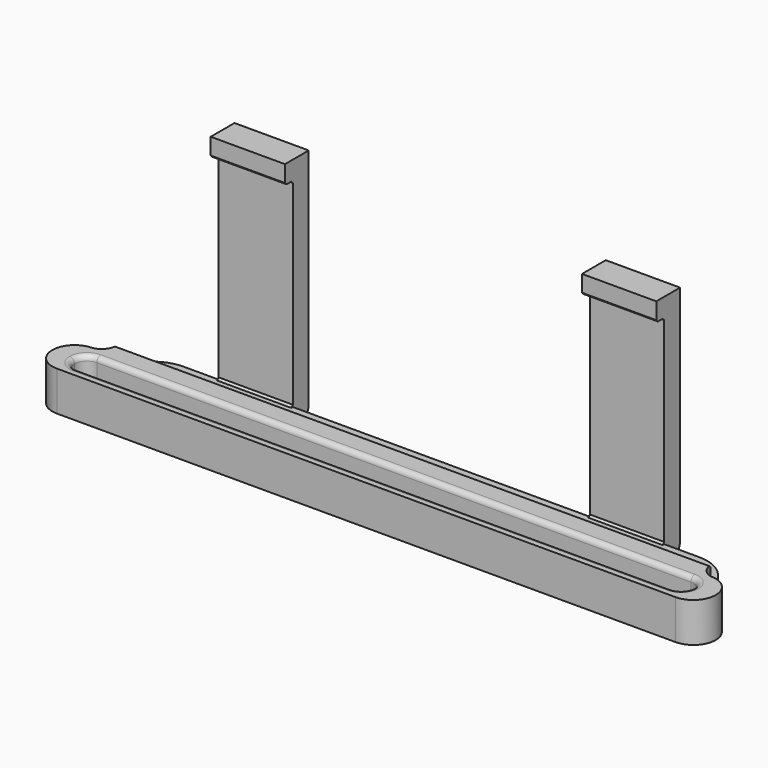
from build123d import *

# Parameters (mm, degrees)
F1_DEPTH    = 8
F2_DEPTH    = 8
F3_DEPTH    = 4
F0_W        = 15
F0_H        = 4
F4_DEPTH    = 48
F5_W        = 15
F5_H        = 3.75
F6_DEPTH    = 2
F7_T1_DEPTH = 43.7732905232
F8_R        = 1
F9_R        = 1
F10_R       = 3
F11_SIZE    = 0.4


# Not quite as in the source:
# - a fillet or chamfer that OpenCascade refuses, or shapes differently, is made with other operations: its cross-section is extruded or revolved along the edge and cut away or added


with BuildPart() as f1:
    # F0 (on Top) → F1 (new body)
    with BuildSketch(Plane.XY):
        with BuildLine():
            Line((60, -5), (-60, -5))
            ThreePointArc((-60, -5), (-61.767766953, -4.267766953), (-62.5, -2.5))
            Line((-62.5, -2.5), (-62.5, -7))
            Line((-62.5, -7), (62.5, -7))
            Line((62.5, -7), (62.5, -2.5))
            ThreePointArc((62.5, -2.5), (61.767766953, -4.267766953), (60, -5))
        make_face()
        with BuildLine():
            Line((62.5, 2), (62.5, -2.5))
            Line((62.5, -2.5), (62.5, -7))
            ThreePointArc((62.5, -7), (67, -2.5), (62.5, 2))
        make_face()
        with BuildLine():
            Line((-62.5, -7), (-62.5, -2.5))
            Line((-62.5, -2.5), (-62.5, 2))
            ThreePointArc((-62.5, 2), (-67, -2.5), (-62.5, -7))
        make_face()
        with BuildLine():
            ThreePointArc((-62.5, -2.5), (-61.767766953, -0.732233047), (-60, 0))
            Line((-60, 0), (60, 0))
            ThreePointArc((60, 0), (61.767766953, -0.732233047), (62.5, -2.5))
            Line((62.5, -2.5), (62.5, 2))
            Line((62.5, 2), (-62.5, 2))
            Line((-62.5, 2), (-62.5, -2.5))
        make_face()
    extrude(amount=F1_DEPTH)

    # F0 (on Top) → F2 (join)
    with BuildSketch(Plane.XY):
        with BuildLine():
            ThreePointArc((-60, 5), (-60.7069250972, 3.047437581), (-62.5, 2))
            Line((-62.5, 2), (62.5, 2))
            ThreePointArc((62.5, 2), (60.7069250972, 3.047437581), (60, 5))
            Line((60, 5), (-60, 5))
        make_face()
    extrude(amount=F2_DEPTH)

    # F0 (on Top) → F3 (join)
    with BuildSketch(Plane.XY):
        Polygon((-60, 12), (-60, 5), (60, 5), (60, 12), (45, 12), (30, 12), (-30, 12), (-45, 12), align=None)
    extrude(amount=F3_DEPTH)

    # F0 (on Top) → F4 (join)
    with BuildSketch(Plane.XY):
        with Locations((-37.5, 14)):
            Rectangle(F0_W, F0_H)
        with Locations((37.5, 14)):
            Rectangle(F0_W, F0_H)
    extrude(amount=F4_DEPTH)

    # F5 (on face) → F6 (join)
    with BuildSketch(Plane.XZ.offset(-12)):
        with Locations((-37.5, 46.125)):
            Rectangle(F5_W, F5_H)
        with Locations((37.5, 46.125)):
            Rectangle(F5_W, F5_H)
    extrude(amount=F6_DEPTH)

    # F7: fillet of radius 8 on 2 edges, made by hand

    # F7_s2 → F7_t1 (cut)
    with BuildSketch(Plane.XY.offset(-19.8866452616)):
        with BuildLine():
            ThreePointArc((52.0453418954, 12), (57.4401609283, 9.9072775118), (60.0125151838, 4.7239819005))
            Line((60.0125151838, 4.7239819005), (60.8092325126, 4.7963800905))
            ThreePointArc((60.8092325126, 4.7963800905), (60.8, 5), (60.8, 12))
            Line((60.8, 12), (60, 12.8))
            Line((60, 12.8), (52.0453418954, 12.8))
            Line((52.0453418954, 12.8), (52.0453418954, 12))
        make_face()
        with BuildLine():
            ThreePointArc((-60.0125151838, 4.7239819005), (-57.4401609283, 9.9072775118), (-52.0453418954, 12))
            Line((-52.0453418954, 12), (-52.0453418954, 12.8))
            Line((-52.0453418954, 12.8), (-60, 12.8))
            Line((-60, 12.8), (-60.8, 12))
            ThreePointArc((-60.8, 12), (-60.8, 5), (-60.8092325126, 4.7963800905))
            Line((-60.8092325126, 4.7963800905), (-60.0125151838, 4.7239819005))
        make_face()
    extrude(amount=F7_T1_DEPTH, mode=Mode.SUBTRACT)

    # F8
    f8_edges = [f1.edges().sort_by_distance(p)[0] for p in [
        (0, 0, 8),
    ]]
    fillet(f8_edges, radius=F8_R)

    # F9
    f9_edges = [f1.edges().sort_by_distance(p)[0] for p in [
        (0, -5, 0),
        (62.5, -2.5, 0),
        (-62.5, -2.5, 0),
        (0, 0, 0),
    ]]
    fillet(f9_edges, radius=F9_R)

    # F10
    f10_edges = [f1.edges().sort_by_distance(p)[0] for p in [
        (-37.5, 16, 0),
        (37.5, 16, 0),
    ]]
    fillet(f10_edges, radius=F10_R)

    # F11
    f11_edges = [f1.edges().sort_by_distance(p)[0] for p in [
        (0, 5, 4),
        (-37.5, 12, 4),
        (37.5, 12, 4),
        (0, 5, 8),
        (37.5, 12, 44.25),
        (-37.5, 12, 44.25),
        (-37.5, 10, 44.25),
        (37.5, 10, 44.25),
    ]]
    chamfer(f11_edges, length=F11_SIZE)


solid = f1.part
